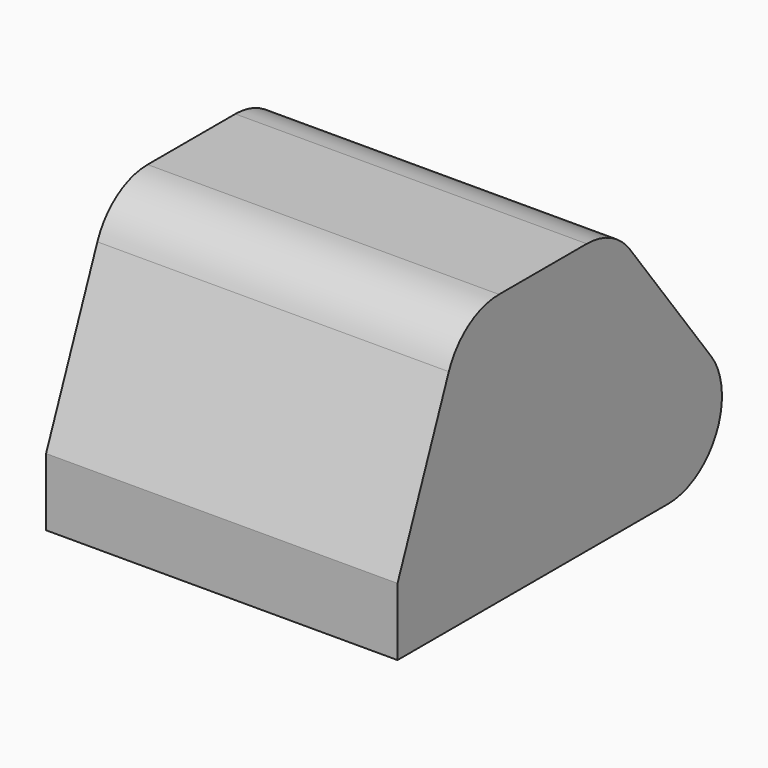
from build123d import *

# Parameters (mm, degrees)
F1_DEPTH = 1300
F2_R     = 500
F3_T     = -6


# Not quite as in the source:
# - a shell that OpenCascade refuses in one call is made with other operations: the cavity is built on its own and cut out


with BuildPart() as f1:
    # F0 (on Right) → F1 (new body, symmetric)
    with BuildSketch(Plane.YZ):
        with BuildLine():
            Line((0, 500), (0, 0))
            Line((0, 0), (2500, 0))
            ThreePointArc((2500, 0), (2947.2135955, 276.39320225), (2900, 800))
            Line((2900, 800), (2000, 2000))
            Line((2000, 2000), (600, 2000))
            Line((600, 2000), (0, 500))
        make_face()
    extrude(amount=F1_DEPTH, both=True)

    # F2
    f2_edges = [f1.edges().sort_by_distance(p)[0] for p in [
        (0, 600, 2000),
        (0, 2000, 2000),
    ]]
    fillet(f2_edges, radius=F2_R)

    # F3: a shell. OpenCascade refuses it in one call, so the cavity is built on its own and cut out:
    # the body offset inwards by the wall thickness, plus a prism from it out through each open face.
    f3_core = offset(f1.part, amount=F3_T, mode=Mode.PRIVATE)
    f3_exits = [f3_core.faces().sort_by_distance(p)[0] for p in [
        (0, 1253, 6),
    ]]
    add(f3_core, mode=Mode.SUBTRACT)
    extrude(f3_exits, amount=-F3_T, mode=Mode.SUBTRACT)


solid = f1.part
